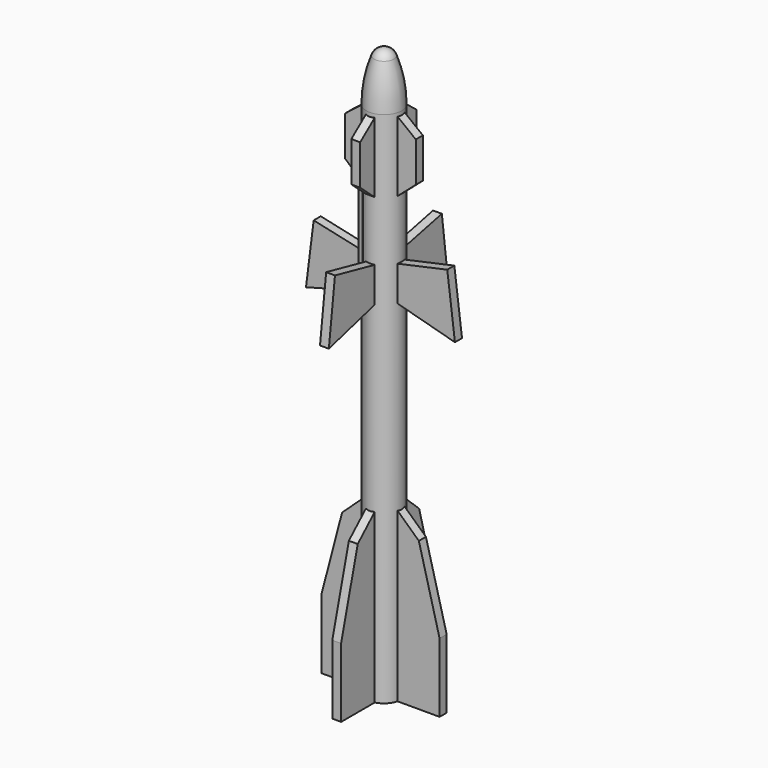
from build123d import *

# Parameters (mm, degrees)
F4_DEPTH     = 0.2
F5_COUNT     = 4
F8_DEPTH     = 6.0416666667
F9_T4_ANGLE  = 67.1804235359
F9_S7_R      = 0.25
F9_T8_DEPTH  = 2
F9_T12_ANGLE = 67.1804235359
F9_S15_R     = 0.25
F9_T16_DEPTH = 2


# Not quite as in the source:
# - a fillet or chamfer that OpenCascade refuses, or shapes differently, is made with other operations: its cross-section is extruded or revolved along the edge and cut away or added


with BuildPart() as f2:
    # F1 (on Front) → F2 (revolve)
    with BuildSketch(Plane.XZ):
        with BuildLine():
            Line((0, 25.6944444444), (0, 0))
            Line((0, 0), (0.7986111111, 0))
            Line((0.7986111111, 0), (0.7986111111, 23.4375))
            ThreePointArc((0.7986111111, 23.4375), (0.7106013269, 24.425281766), (0.4493446353, 25.3819444444))
            ThreePointArc((0.4493446353, 25.3819444444), (0.2736635029, 25.6086390085), (0, 25.6944444444))
        make_face()
    revolve(axis=Axis((0, 0, 12.8472222222), (0, 0, 1)))

    # F3 (on Front) → F4 (join, symmetric)
    with BuildSketch(Plane.XZ):
        Polygon((0, 23.8888888889), (0, 0), (0.7986111111, 0), (2.6736111111, 0), (2.6736111111, 3.125), (1.7361111111, 6.7013888889), (0.4, 7.9385288066), (0.4, 15.9410660661), (3.3680555556, 15.1388888889), (3.0208333333, 17.9166666667), (0.4, 17.343359375), (0.4, 19.7922705314), (1.5972222222, 20.8333333333), (1.5972222222, 22.6388888889), align=None)
    extrude(amount=F4_DEPTH, both=True)

    # F5: F2 ×4 about axis
    f5_axis = Axis((0, 0, 0), (0, 0, 1))


with BuildPart() as f2_1:
    add(f2.part)
    for i in range(1, F5_COUNT):
        add(f2.part.rotate(f5_axis, i * 360 / F5_COUNT))

    # F7 (on offset) → F8 (join)
    with BuildSketch(Plane.XY.offset(15.4166666667)):
        with BuildLine():
            Line((-0.4086259328, -0.7035839656), (-0.1424359704, -0.4373940032))
            Line((-0.1424359704, -0.4373940032), (-0.4373940032, -0.1424359704))
            Line((-0.4373940032, -0.1424359704), (-0.7035839656, -0.4086259328))
            ThreePointArc((-0.7035839656, -0.4086259328), (-0.6354140103, -0.6354140103), (-0.4086259328, -0.7035839656))
        make_face()
    extrude(amount=F8_DEPTH)

    # F9: chamfer of 0.1 on 2 edges, made by hand


with BuildPart() as f9_tool2:
    # F9_s3 → F9_t4 (revolve)
    with BuildSketch(Plane(origin=(0, 0, 0), x_dir=(0, 0, 1), z_dir=(-0.197824804, 0.9802373932, 0))):
        Polygon((21.5583333333, -0.7986111111), (21.4583333333, -0.8986111111), (21.4583333333, -0.7986111111), align=None)
    revolve(axis=Axis((0, 0, 21.4583333333), (0, 0, 1)), revolution_arc=F9_T4_ANGLE)

    split(bisect_by=Plane(origin=(0.1474790164, -0.1474790164, 0), x_dir=(0, 0, 1), z_dir=(-0.7071067812, 0.7071067812, 0)), keep=Keep.TOP)

    split(bisect_by=Plane(origin=(-0.1474790164, 0.1474790164, 0), x_dir=(0, 0, 1), z_dir=(0.7071067812, -0.7071067812, 0)), keep=Keep.TOP)

    # F9_s7 → F9_t8 (intersect, symmetric)
    with BuildSketch(Plane.XY.offset(21.5)):
        with Locations((-0.458637315, -0.458637315)):
            Circle(F9_S7_R)
    extrude(amount=F9_T8_DEPTH, both=True, mode=Mode.INTERSECT)


with BuildPart() as f2_2:
    add(f2_1.part)

    # F9_t1: union F9_tool2
    add(f9_tool2.part)


with BuildPart() as f9_tool10:
    # F9_s11 → F9_t12 (revolve)
    with BuildSketch(Plane(origin=(0, 0, 0), x_dir=(0, 0, 1), z_dir=(-0.197824804, 0.9802373932, 0))):
        Polygon((15.3166666667, -0.7986111111), (15.4166666667, -0.8986111111), (15.4166666667, -0.7986111111), align=None)
    revolve(axis=Axis((0, 0, 15.4166666667), (0, 0, 1)), revolution_arc=F9_T12_ANGLE)

    split(bisect_by=Plane(origin=(0.1474790164, -0.1474790164, 0), x_dir=(0, 0, 1), z_dir=(-0.7071067812, 0.7071067812, 0)), keep=Keep.TOP)

    split(bisect_by=Plane(origin=(-0.1474790164, 0.1474790164, 0), x_dir=(0, 0, 1), z_dir=(0.7071067812, -0.7071067812, 0)), keep=Keep.TOP)

    # F9_s15 → F9_t16 (intersect, symmetric)
    with BuildSketch(Plane.XY.offset(15.4)):
        with Locations((-0.458637315, -0.458637315)):
            Circle(F9_S15_R)
    extrude(amount=F9_T16_DEPTH, both=True, mode=Mode.INTERSECT)


with BuildPart() as f2_3:
    add(f2_2.part)

    # F9_t9: union F9_tool10
    add(f9_tool10.part)


solid = f2_3.part
